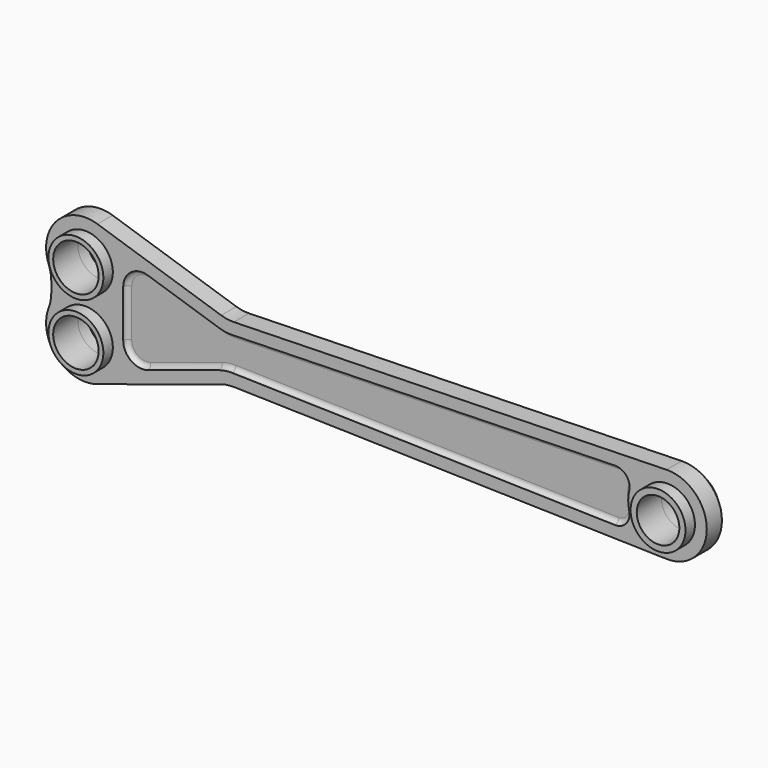
from build123d import *

# Parameters (mm, degrees)
F0_R          = 29
F1_DEPTH      = 20
F3_DEPTH      = 5
F5_DEPTH      = 5
F6_R          = 4.99999
F7_R          = 4.99999
F8_R          = 29
F8_R_2        = 22.5
F8_R_3        = 24
F9_DEPTH      = 12.5
F9_DEPTH_BACK = 32.5


# Not quite as in the source:
# - a fillet or chamfer is up to 0.001 mm smaller than in the source, because OpenCascade refuses the exact size


with BuildPart() as f1:
    # F0 (on Front) → F1 (new body)
    with BuildSketch(Plane.XZ):
        with BuildLine():
            Line((228.5028561992, 32.1062064806), (97.7975828549, 74.4774856478))
            ThreePointArc((97.7975828549, 74.4774856478), (54.8450921386, 63.5119541924), (46.3006134969, 20.0130895684))
            ThreePointArc((46.3006134969, 20.0130895684), (48.3193625322, 12.9155090118), (49, 5.5678746945))
            Line((49, 5.5678746945), (49, -5.5678746945))
            ThreePointArc((49, -5.5678746945), (48.3193625322, -12.9155090118), (46.3006134969, -20.0130895684))
            ThreePointArc((46.3006134969, -20.0130895684), (54.8450921386, -63.5119541924), (97.7975828549, -74.4774856478))
            Line((97.7975828549, -74.4774856478), (228.5028561992, -32.1062064806))
            ThreePointArc((228.5028561992, -32.1062064806), (235.0832865864, -30.5729005697), (241.8279137151, -30.1690491218))
            Line((241.8279137151, -30.1690491218), (698.9728356822, -41.4872864076))
            ThreePointArc((698.9728356822, -41.4872864076), (741.5, 0), (698.9728356822, 41.4872864076))
            Line((698.9728356822, 41.4872864076), (241.8279137151, 30.1690491218))
            ThreePointArc((241.8279137151, 30.1690491218), (235.0832865864, 30.5729005697), (228.5028561992, 32.1062064806))
        make_face()
        with Locations((85, -35)):
            Circle(F0_R, mode=Mode.SUBTRACT)
        with Locations((85, 35)):
            Circle(F0_R, mode=Mode.SUBTRACT)
        with Locations((700, 0)):
            Circle(F0_R, mode=Mode.SUBTRACT)
    extrude(amount=F1_DEPTH)

    # F2 (on face) → F3 (cut)
    with BuildSketch(Plane.XZ.offset(20)):
        with BuildLine():
            ThreePointArc((659.5520018106, -9.2849040098), (658.5, 0), (659.5520018106, 9.2849040098))
            ThreePointArc((659.5520018106, 9.2849040098), (656.5489690059, 22.1304501377), (644.5609792177, 27.6362981366))
            Line((644.5609792177, 27.6362981366), (240.0035775219, 17.6200506665))
            ThreePointArc((240.0035775219, 17.6200506665), (233.2589503932, 18.0239021144), (226.678520006, 19.5572080254))
            Line((226.678520006, 19.5572080254), (151.1675098096, 44.0359303551))
            ThreePointArc((151.1675098096, 44.0359303551), (133.238839262, 41.1870107565), (125, 25.010636067))
            Line((125, 25.010636067), (125, -25.010636067))
            ThreePointArc((125, -25.010636067), (133.238839262, -41.1870107565), (151.1675098096, -44.0359303551))
            Line((151.1675098096, -44.0359303551), (226.678520006, -19.5572080254))
            ThreePointArc((226.678520006, -19.5572080254), (233.2589503932, -18.0239021144), (240.0035775219, -17.6200506665))
            Line((240.0035775219, -17.6200506665), (644.5609792177, -27.6362981366))
            ThreePointArc((644.5609792177, -27.6362981366), (656.5489690059, -22.1304501377), (659.5520018106, -9.2849040098))
        make_face()
    extrude(amount=-F3_DEPTH, mode=Mode.SUBTRACT)

    # F4 (on face) → F5 (cut)
    with BuildSketch(Plane(origin=(0, 0, 0), x_dir=(-1, 0, 0), z_dir=(0, 1, 0))):
        with BuildLine():
            ThreePointArc((-659.5520018106, 9.2849040098), (-658.5, 0), (-659.5520018106, -9.2849040098))
            ThreePointArc((-659.5520018106, -9.2849040098), (-656.5489690059, -22.1304501377), (-644.5609792177, -27.6362981366))
            Line((-644.5609792177, -27.6362981366), (-240.0035775219, -17.6200506665))
            ThreePointArc((-240.0035775219, -17.6200506665), (-233.2589503932, -18.0239021144), (-226.678520006, -19.5572080254))
            Line((-226.678520006, -19.5572080254), (-151.1675098096, -44.0359303551))
            ThreePointArc((-151.1675098096, -44.0359303551), (-133.238839262, -41.1870107565), (-125, -25.010636067))
            Line((-125, -25.010636067), (-125, 25.010636067))
            ThreePointArc((-125, 25.010636067), (-133.238839262, 41.1870107565), (-151.1675098096, 44.0359303551))
            Line((-151.1675098096, 44.0359303551), (-226.678520006, 19.5572080254))
            ThreePointArc((-226.678520006, 19.5572080254), (-233.2589503932, 18.0239021144), (-240.0035775219, 17.6200506665))
            Line((-240.0035775219, 17.6200506665), (-644.5609792177, 27.6362981366))
            ThreePointArc((-644.5609792177, 27.6362981366), (-656.5489690059, 22.1304501377), (-659.5520018106, 9.2849040098))
        make_face()
    extrude(amount=-F5_DEPTH, mode=Mode.SUBTRACT)

    # F6 (radius 5 in the source; OpenCascade refuses exactly that, so slightly less here)
    f6_edges = [f1.edges().sort_by_distance(p)[0] for p in [
        (442.282278, -15, 22.628174),
    ]]
    fillet(f6_edges, radius=F6_R)

    # F7 (radius 5 in the source; OpenCascade refuses exactly that, so slightly less here)
    f7_edges = [f1.edges().sort_by_distance(p)[0] for p in [
        (442.282278, -5, 22.628174),
    ]]
    fillet(f7_edges, radius=F7_R)

    # F8 (on face) → F9 (join, two sides)
    with BuildSketch(Plane(origin=(0, 0, 0), x_dir=(-1, 0, 0), z_dir=(0, 1, 0))) as f9_sk:
        with Locations((-700, 0)):
            Circle(F8_R)
        with Locations((-700, 0)):
            Circle(F8_R_2, mode=Mode.SUBTRACT)
        with Locations((-85, 35)):
            Circle(F8_R)
        with Locations((-85, 35)):
            Circle(F8_R_3, mode=Mode.SUBTRACT)
        with Locations((-85, -35)):
            Circle(F8_R)
        with Locations((-85, -35)):
            Circle(F8_R_3, mode=Mode.SUBTRACT)
    extrude(amount=F9_DEPTH)
    extrude(f9_sk.sketch, amount=-F9_DEPTH_BACK)


solid = f1.part
